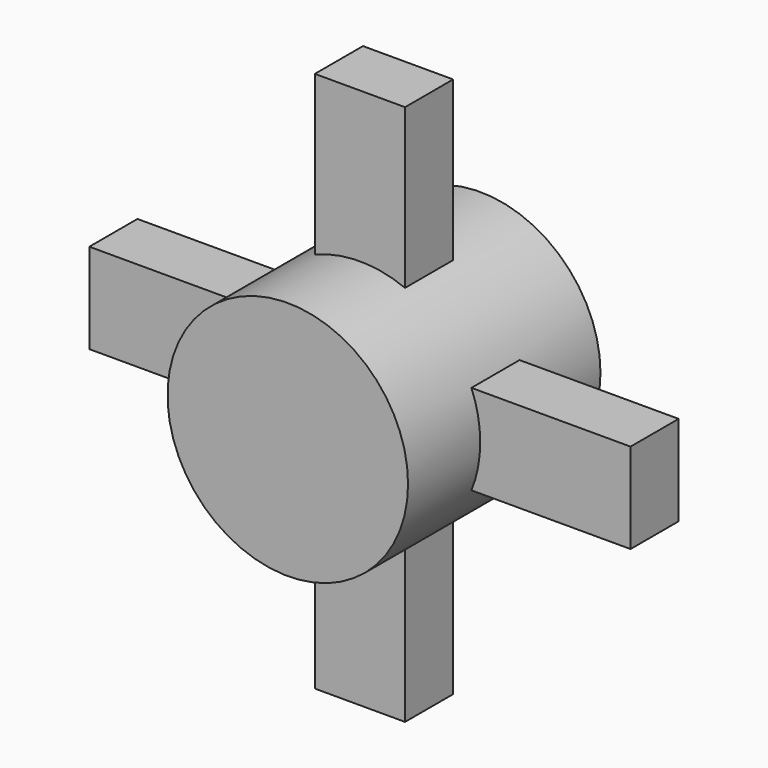
from build123d import *

# Parameters (mm, degrees)
F0_R            = 20
F1_DEPTH        = 20
F3_W            = 15
F3_H            = 10
F4_DEPTH        = 30
F4_COPIES_COUNT = 4


# Not quite as in the source:
# - a pattern or mirror of a feature is missing from the dataset's text; its kind, count and spacing are read off the source's solid


with BuildPart() as f1:
    # F0 (on Front) → F1 (new body, symmetric)
    with BuildSketch(Plane.XZ):
        Circle(F0_R)
    extrude(amount=F1_DEPTH, both=True)

    # F3 (on offset) → F4 (join)
    with BuildSketch(Plane.XY.offset(15)):
        Rectangle(F3_W, F3_H)
    f4 = extrude(amount=F4_DEPTH)

    # F4_copies: F4 ×4 about axis
    f4_copies_axis = Axis((0, 0, 0), (0, 1, 0))
    for i in range(1, F4_COPIES_COUNT):
        add(f4.rotate(f4_copies_axis, i * 360 / F4_COPIES_COUNT))


solid = f1.part
